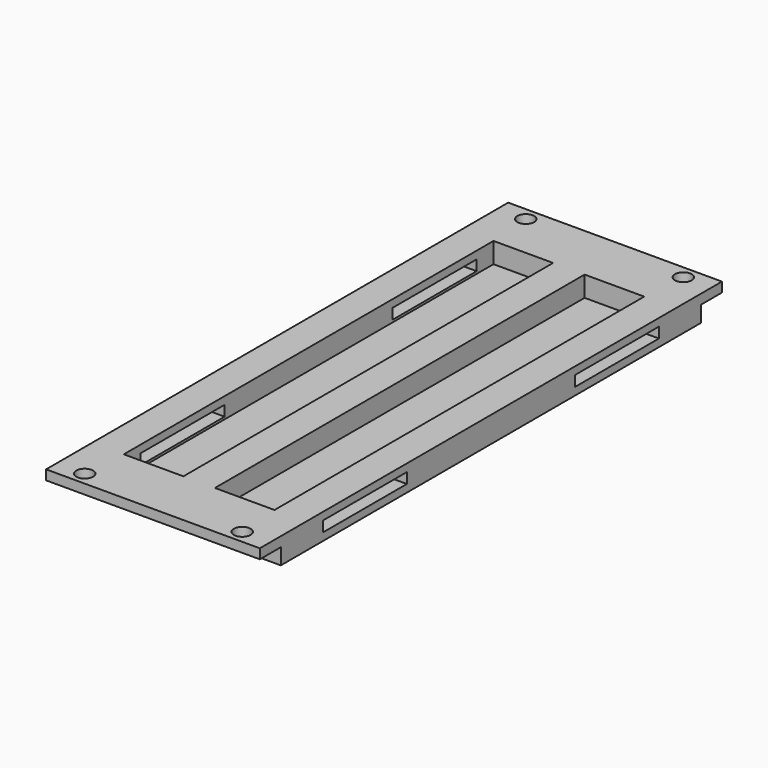
from build123d import *

# Parameters (mm, degrees)
F0_W      = 40.7
F0_H      = 100
F1_DEPTH  = 1
F2_W      = 40.7
F2_H      = 100
F2_W_2    = 6
F2_H_2    = 88
F3_DEPTH  = 3.9
F4_W      = 40.7
F4_H      = 1.85
F5_DEPTH  = 5
F6_R      = 1.6
F7_DEPTH  = 1.851
F8_W      = 20
F8_H      = 2
F9_DEPTH  = 6
F10_W     = 20
F10_H     = 2
F11_DEPTH = 6


# Not quite as in the source:
# - a pattern or mirror of a feature is missing from the dataset's text; its kind, count and spacing are read off the source's solid


with BuildPart() as f1:
    # F0 (on Top) → F1 (new body)
    with BuildSketch(Plane.XY):
        Rectangle(F0_W, F0_H)
    extrude(amount=-F1_DEPTH)

    # F2 (on Top) → F3 (join)
    with BuildSketch(Plane.XY):
        Rectangle(F2_W, F2_H)
        Polygon((-14.35, -44), (-14.35, 44), (-3, 44), (3, 44), (14.35, 44), (14.35, -44), (3, -44), (-3, -44), align=None, mode=Mode.SUBTRACT)
        Rectangle(F2_W_2, F2_H_2)
    extrude(amount=F3_DEPTH)

    # F4 (on face) → F5 (join)
    with BuildSketch(Plane.XZ.offset(50)):
        with Locations((0, 2.975)):
            Rectangle(F4_W, F4_H)
    f5 = extrude(amount=F5_DEPTH)

    # F5_copies: F5 across plane
    add(f5.mirror(Plane.ZX))

    # F6 (on face) → F7 (cut, through all)
    with BuildSketch(Plane(origin=(0, 0, 2.05), x_dir=(1, 0, 0), z_dir=(0, 0, -1))):
        with Locations((-15, 52.5)):
            Circle(F6_R)
        with Locations((15, 52.5)):
            Circle(F6_R)
        with Locations((-15, -52.5)):
            Circle(F6_R)
        with Locations((15, -52.5)):
            Circle(F6_R)
    extrude(amount=-F7_DEPTH, mode=Mode.SUBTRACT)

    # F8 (on face) → F9 (cut, through all)
    with BuildSketch(Plane(origin=(-20.35, 0, 0), x_dir=(0, -1, 0), z_dir=(-1, 0, 0))):
        with Locations((-30, 1.45)):
            Rectangle(F8_W, F8_H)
        with Locations((30, 1.45)):
            Rectangle(F8_W, F8_H)
    extrude(amount=-F9_DEPTH, mode=Mode.SUBTRACT)

    # F10 (on face) → F11 (cut, through all)
    with BuildSketch(Plane.YZ.offset(20.35)):
        with Locations((-30, 1.45)):
            Rectangle(F10_W, F10_H)
        with Locations((30, 1.45)):
            Rectangle(F10_W, F10_H)
    extrude(amount=-F11_DEPTH, mode=Mode.SUBTRACT)


solid = f1.part
